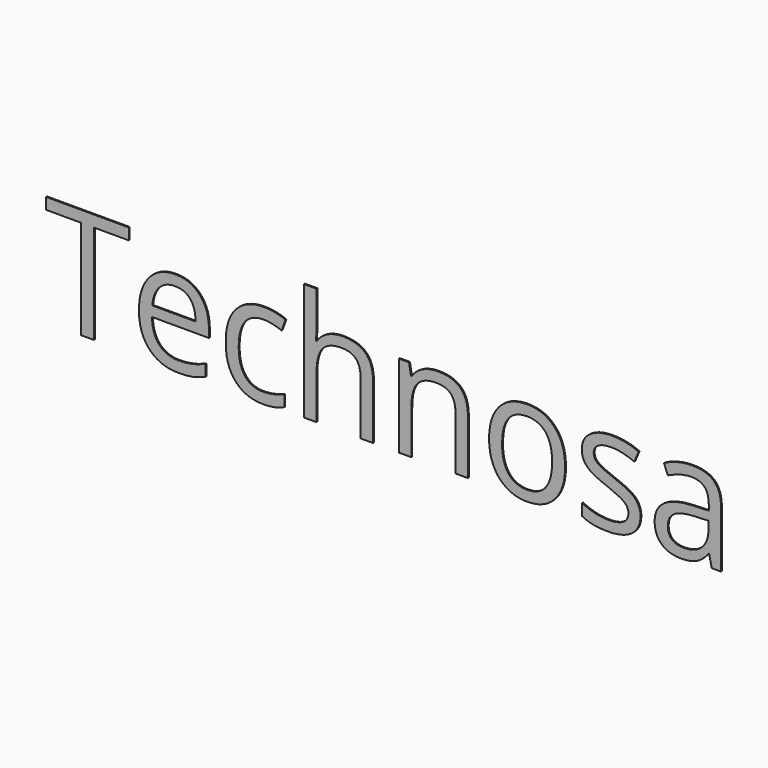
from build123d import *

# Parameters (mm, degrees)
F0_TEXT_SIZE = 34.7075375935
F1_DEPTH     = 0.254


# Not quite as in the source:
# - Text() gives the source's letters only with a copy of the font that has no kerning and outlines rounded to 1/6400 em; it was checked with that copy


with BuildPart() as f1:
    # F0 (on Front) → F1 (new body)
    with BuildSketch(Plane.XZ):
        with Locations((-63.5695904493, 5.1513258368)):
            Text('Technosa', F0_TEXT_SIZE, font='Open Sans', text_align=(TextAlign.LEFT, TextAlign.BOTTOM))
    extrude(amount=F1_DEPTH)


solid = f1.part
